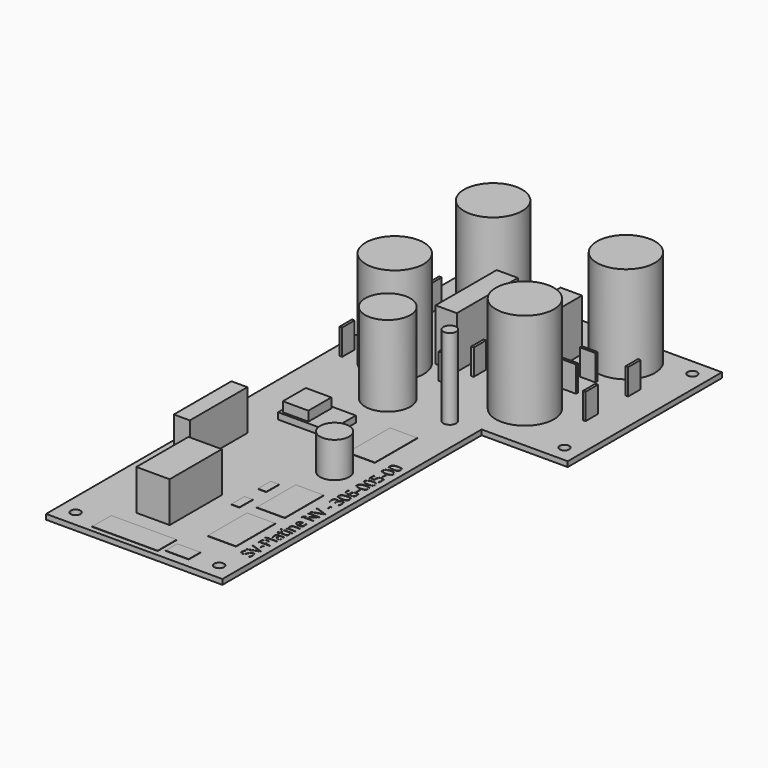
from build123d import *

# Parameters (mm, degrees)
F0_R         = 1.5
F1_DEPTH     = 1.6
F2_TEXT_SIZE = 4.8621135
F3_DEPTH     = 0.1
F4_R         = 9
F5_DEPTH     = 30
F4_R_2       = 7
F6_DEPTH     = 25
F4_W         = 6.6660640296
F4_H         = 23.4645446762
F4_W_2       = 6.5771816298
F4_H_2       = 23.6423034221
F7_DEPTH     = 16
F4_W_3       = 0.8
F4_H_3       = 4.8
F4_W_4       = 4.8
F4_H_4       = 1.0472461581
F4_H_5       = 0.8
F8_DEPTH     = 8
F4_W_5       = 4.9606468529
F4_H_6       = 22.2835317254
F4_W_6       = 10.3101776913
F4_H_7       = 20.1759487391
F9_DEPTH     = 12.5
F4_R_3       = 4.5
F10_DEPTH    = 11
F4_R_4       = 2
F11_DEPTH    = 25
F4_W_7       = 7.9103969038
F4_H_8       = 8.8880844414
F12_DEPTH    = 5
F4_W_8       = 15.7319093123
F4_H_9       = 10.3990584612
F13_DEPTH    = 2
F4_W_9       = 8.7992027402
F4_H_10      = 15.2875036001
F4_W_10      = 8.7103224359
F4_H_11      = 15.1097476482
F4_W_11      = 7.1993487654
F4_H_12      = 4.5329257846
F4_W_12      = 20.2648309059
F4_H_13      = 7.3771029711
F4_W_13      = 8.4760577884
F4_H_14      = 16.4451003075
F4_W_14      = 4.6566370875
F4_H_15      = 4.7195702791
F4_W_15      = 2.5775446557
F4_H_16      = 5.1550939679
F4_W_16      = 2.598434221
F4_H_17      = 4.9606487155
F14_DEPTH    = 0.1


# Not quite as in the source:
# - a feature names something its author has since deleted; it is built from what else it names
# - Text() gives the source's letters only with a copy of the font that has no kerning and outlines rounded to 1/6400 em; it was checked with that copy


with BuildPart() as f1:
    # F0 (on Top) → F1 (new body)
    with BuildSketch(Plane.XY):
        Polygon((13.97, -29.845), (40.64, -29.845), (40.64, 29.845), (-40.64, 29.845), (-40.64, -29.845), (-40.64, -130.175), (13.97, -130.175), align=None)
        with Locations((-35.56, -125.095)):
            Circle(F0_R, mode=Mode.SUBTRACT)
        with Locations((8.89, -125.095)):
            Circle(F0_R, mode=Mode.SUBTRACT)
        with Locations((-35.56, 24.765)):
            Circle(F0_R, mode=Mode.SUBTRACT)
        with Locations((35.56, -24.765)):
            Circle(F0_R, mode=Mode.SUBTRACT)
        with Locations((35.56, 24.765)):
            Circle(F0_R, mode=Mode.SUBTRACT)
    extrude(amount=-F1_DEPTH)

    # F2 (on face) → F3 (cut)
    with BuildSketch(Plane.XY):
        with Locations(Location((12.2062923127, -117.3487902395), (0, 0, 90))):
            Text('SV-Platine NV - 306-005-00', F2_TEXT_SIZE, font='Open Sans', text_align=(TextAlign.LEFT, TextAlign.BOTTOM))
    extrude(amount=-F3_DEPTH, mode=Mode.SUBTRACT)

    # F4 (on face) → F5 (join)
    with BuildSketch(Plane.XY):
        with Locations((19.2125588655, 19.46840249)):
            Circle(F4_R)
        with Locations((-22.8230375797, 20.601099357)):
            Circle(F4_R)
        with Locations((-24.0658465773, -15.9294046462)):
            Circle(F4_R)
        with Locations((15.3110502288, -14.7641794756)):
            Circle(F4_R)
    extrude(amount=F5_DEPTH)

    # F4 (on face) → F6 (join)
    with BuildSketch(Plane.XY):
        with Locations((-13.9148654416, -31.3201807439)):
            Circle(F4_R_2)
    extrude(amount=F6_DEPTH)

    # F4 (on face) → F7 (join)
    with BuildSketch(Plane.XY):
        with Locations((4.9861661391, 4.3562897481)):
            Rectangle(F4_W, F4_H)
        with Locations((-12.8344432451, 1.7787441611)):
            Rectangle(F4_W_2, F4_H_2)
    extrude(amount=F7_DEPTH)

    # F4 (on face) → F8 (join)
    with BuildSketch(Plane.XY):
        with Locations((-34.1095917583, 11.9121420406)):
            Rectangle(F4_W_3, F4_H_3)
        with Locations((-34.1095917583, -3.3560573332)):
            Rectangle(F4_W_3, F4_H_3)
        with Locations((-36.4932448328, -18.849787882)):
            Rectangle(F4_W_3, F4_H_3)
        with Locations((-5.1127972737, -7.1121087506)):
            Rectangle(F4_W_3, F4_H_3)
        with Locations((-7.6792319305, -15.8933605999)):
            Rectangle(F4_W_4, F4_H_4)
        with Locations((17.7642963827, -0.6118016317)):
            Rectangle(F4_W_4, F4_H_5)
        with Locations((30.5019300431, -8.3487350494)):
            Rectangle(F4_W_3, F4_H_3)
        with Locations((17.7013929933, 6.9678770378)):
            Rectangle(F4_W_4, F4_H_5)
        with Locations((30.4704792798, 8.1630134955)):
            Rectangle(F4_W_3, F4_H_3)
        with Locations((-5.0379939102, 17.0493846551)):
            Rectangle(F4_W_3, F4_H_3)
    extrude(amount=F8_DEPTH)

    # F4 (on face) → F9 (join)
    with BuildSketch(Plane.XY):
        with Locations((-31.5601835027, -77.828604728)):
            Rectangle(F4_W_5, F4_H_6)
        with Locations((-18.7894604169, -106.0111671686)):
            Rectangle(F4_W_6, F4_H_7)
    extrude(amount=F9_DEPTH)

    # F4 (on face) → F10 (join)
    with BuildSketch(Plane.XY):
        with Locations((0, -69.3040192127)):
            Circle(F4_R_3)
    extrude(amount=F10_DEPTH)

    # F4 (on face) → F11 (join)
    with BuildSketch(Plane.XY):
        with Locations((5.2083665505, -31.1960484833)):
            Circle(F4_R_4)
    extrude(amount=F11_DEPTH)

    # F4 (on face) → F12 (join)
    with BuildSketch(Plane.XY):
        with Locations((-22.833539173, -51.3938907534)):
            Rectangle(F4_W_7, F4_H_8)
    extrude(amount=F12_DEPTH)

    # F4 (on face) → F13 (join)
    with BuildSketch(Plane.XY):
        with Locations((-19.8115906678, -51.3494499028)):
            Rectangle(F4_W_8, F4_H_9)
        with Locations((-22.833539173, -51.3938907534)):
            Rectangle(F4_W_7, F4_H_8, mode=Mode.SUBTRACT)
    extrude(amount=F13_DEPTH)

    # F4 (on face) → F14 (join)
    with BuildSketch(Plane.XY):
        with Locations((1.5198118053, -107.2267740965)):
            Rectangle(F4_W_9, F4_H_10)
        with Locations((1.4753716532, -88.2951542735)):
            Rectangle(F4_W_10, F4_H_11)
        with Locations((-2.3909449228, -125.009778887)):
            Rectangle(F4_W_11, F4_H_12)
        with Locations((-17.5451280084, -124.8320117593)):
            Rectangle(F4_W_12, F4_H_13)
        with Locations((0.5259342724, -51.4144152403)):
            Rectangle(F4_W_13, F4_H_14)
        with Locations((-30.2486522123, -93.2639464736)):
            Rectangle(F4_W_14, F4_H_15)
        with Locations((-7.4571531732, -95.8343036473)):
            Rectangle(F4_W_15, F4_H_16)
        with Locations((-7.4656188954, -85.5451636016)):
            Rectangle(F4_W_16, F4_H_17)
    extrude(amount=F14_DEPTH)


solid = f1.part
